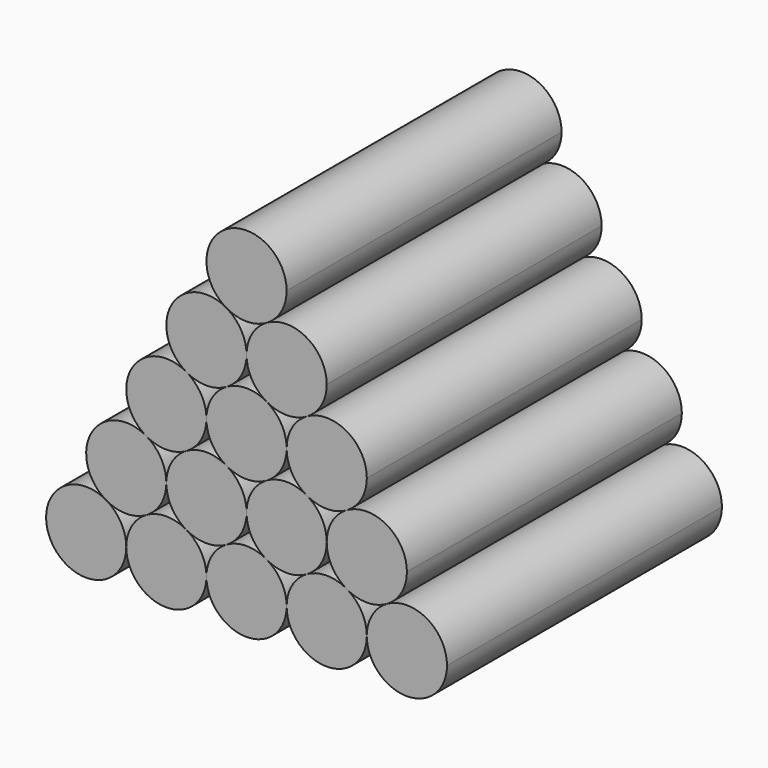
from build123d import *

# Parameters (mm, degrees)
F1_DEPTH = 76.2


# Not quite as in the source:
# - a feature names something its author has since deleted; it is built from what else it names


with BuildPart() as f1:
    # F0 (on Front) → F1 (new body)
    with BuildSketch(Plane.XZ):
        with BuildLine():
            ThreePointArc((-13.3350000199, 23.0968975304), (-25.4789658129, 19.8429317256), (-22.2250001126, 7.6989659046))
            ThreePointArc((-22.2250001126, 7.6989659046), (-17.780000037, 6.5079316793), (-13.3349999515, 7.6989658677))
            ThreePointArc((-13.3349999515, 7.6989658677), (-10.0810341464, 10.9529317035), (-8.89, 15.3979316793))
            ThreePointArc((-8.89, 15.3979316793), (-10.0810341661, 19.8429316893), (-13.3350000199, 23.0968975304))
        make_face()
    extrude(amount=F1_DEPTH)


with BuildPart() as f1b:
    # F0 (on Front) → F1, piece 2 (new body)
    with BuildSketch(Plane.XZ):
        with BuildLine():
            ThreePointArc((-8.89, 15.3979316793), (-7.6989658311, 10.9529316645), (-4.4449999705, 7.6989658226))
            ThreePointArc((-4.4449999705, 7.6989658226), (6.75e-08, 6.5079316793), (4.4450000875, 7.6989658901))
            ThreePointArc((4.4450000875, 7.6989658901), (7.6989658649, 10.952931723), (8.89, 15.3979316793))
            ThreePointArc((8.89, 15.3979316793), (7.6989657927, 19.8429317606), (4.4449998375, 23.0968976128))
            ThreePointArc((4.4449998375, 23.0968976128), (-4.81e-08, 24.2879316793), (-4.4449999207, 23.0968975647))
            ThreePointArc((-4.4449999207, 23.0968975647), (-7.6989658168, 19.8429317189), (-8.89, 15.3979316793))
        make_face()
    extrude(amount=F1_DEPTH)


with BuildPart() as f1c:
    # F0 (on Front) → F1, piece 3 (new body)
    with BuildSketch(Plane.XZ):
        with BuildLine():
            ThreePointArc((8.89, 15.3979316793), (10.0810341244, 10.9529317415), (13.3349998755, 7.6989659115))
            ThreePointArc((13.3349998755, 7.6989659115), (17.7799998064, 6.5079316793), (22.2249997892, 7.6989657179))
            ThreePointArc((22.2249997892, 7.6989657179), (25.4789657788, 10.9529315739), (26.67, 15.3979316793))
            ThreePointArc((26.67, 15.3979316793), (22.2250001076, 23.0968974568), (13.3350002151, 23.0968976431))
            ThreePointArc((13.3350002151, 23.0968976431), (10.0810342225, 19.8429317869), (8.89, 15.3979316793))
        make_face()
    extrude(amount=F1_DEPTH)


with BuildPart() as f1d:
    # F0 (on Front) → F1, piece 4 (new body)
    with BuildSketch(Plane.XZ):
        with BuildLine():
            ThreePointArc((22.2249997892, 7.6989657179), (18.9710340995, 4.4449998946), (17.78, 0))
            ThreePointArc((17.78, 0), (18.9710341607, -4.4450000007), (22.2250000013, -7.6989658404))
            ThreePointArc((22.2250000013, -7.6989658404), (26.6699999179, -8.89), (31.1149998565, -7.6989659225))
            ThreePointArc((31.1149998565, -7.6989659225), (34.3689657982, -4.4450000718), (35.56, 0))
            ThreePointArc((35.56, 0), (31.1149998946, 7.6989659005), (22.2249997892, 7.6989657179))
        make_face()
    extrude(amount=F1_DEPTH)


with BuildPart() as f1e:
    # F0 (on Front) → F1, piece 5 (new body)
    with BuildSketch(Plane.XZ):
        with BuildLine():
            ThreePointArc((4.4450000875, 7.6989658901), (1.1910341856, 4.4450000437), (0, 0))
            ThreePointArc((0, 0), (1.191034094, -4.4449998851), (4.4449997703, -7.698965707))
            ThreePointArc((4.4449997703, -7.698965707), (8.8899998666, -8.89), (13.3349999987, -7.6989658404))
            ThreePointArc((13.3349999987, -7.6989658404), (16.5889658393, -4.4450000007), (17.78, 0))
            ThreePointArc((17.78, 0), (16.5889658037, 4.4450000622), (13.3349998755, 7.6989659115))
            ThreePointArc((13.3349998755, 7.6989659115), (8.8899999786, 8.89), (4.4450000875, 7.6989658901))
        make_face()
    extrude(amount=F1_DEPTH)


with BuildPart() as f1f:
    # F0 (on Front) → F1, piece 6 (new body)
    with BuildSketch(Plane.XZ):
        with BuildLine():
            ThreePointArc((-13.3349999515, 7.6989658677), (-16.5889658256, 4.4450000243), (-17.78, 0))
            ThreePointArc((-17.78, 0), (-16.5889664254, -4.4449989854), (-13.3350020292, -7.6989646681))
            ThreePointArc((-13.3350020292, -7.6989646681), (-8.8900010389, -8.89), (-4.4449997703, -7.698965707))
            ThreePointArc((-4.4449997703, -7.698965707), (-1.191034094, -4.4449998851), (0, 0))
            ThreePointArc((0, 0), (-1.1910341518, 4.4449999853), (-4.4449999705, 7.6989658226))
            ThreePointArc((-4.4449999705, 7.6989658226), (-8.889999955, 8.89), (-13.3349999515, 7.6989658677))
        make_face()
    extrude(amount=F1_DEPTH)


with BuildPart() as f1g:
    # F0 (on Front) → F1, piece 7 (new body)
    with BuildSketch(Plane.XZ):
        with BuildLine():
            ThreePointArc((-22.2249979726, -7.6989646691), (-18.9710335751, -4.4449989863), (-17.78, 0))
            ThreePointArc((-17.78, 0), (-18.9710341928, 4.4450000563), (-22.2250001126, 7.6989659046))
            ThreePointArc((-22.2250001126, 7.6989659046), (-34.3689658547, 4.4449999739), (-31.1150000603, -7.6989658048))
            ThreePointArc((-31.1150000603, -7.6989658048), (-26.6699988643, -8.89), (-22.2249979726, -7.6989646691))
        make_face()
    extrude(amount=F1_DEPTH)


with BuildPart() as f1h:
    # F0 (on Front) → F1, piece 8 (new body)
    with BuildSketch(Plane.XZ):
        with BuildLine():
            ThreePointArc((-26.67, -15.3979316793), (-27.8610341778, -10.9529316492), (-31.1150000603, -7.6989658048))
            ThreePointArc((-31.1150000603, -7.6989658048), (-43.2589658414, -10.9529316824), (-40.0050000541, -23.0968974877))
            ThreePointArc((-40.0050000541, -23.0968974877), (-35.559998118, -24.2879316793), (-31.1149966862, -23.0968956057))
            ThreePointArc((-31.1149966862, -23.0968956057), (-27.8610332037, -19.8429300224), (-26.67, -15.3979316793))
        make_face()
    extrude(amount=F1_DEPTH)


with BuildPart() as f1i:
    # F0 (on Front) → F1, piece 9 (new body)
    with BuildSketch(Plane.XZ):
        with BuildLine():
            ThreePointArc((-13.3350020292, -7.6989646681), (-17.780000001, -6.5079316793), (-22.2249979726, -7.6989646691))
            ThreePointArc((-22.2249979726, -7.6989646691), (-25.4789652544, -10.9529306656), (-26.67, -15.3979316793))
            ThreePointArc((-26.67, -15.3979316793), (-25.4789658625, -19.8429316396), (-22.2250000793, -23.0968974731))
            ThreePointArc((-22.2250000793, -23.0968974731), (-17.7799999131, -24.2879316793), (-13.3349997703, -23.0968973863))
            ThreePointArc((-13.3349997703, -23.0968973863), (-10.081034094, -19.8429315644), (-8.89, -15.3979316793))
            ThreePointArc((-8.89, -15.3979316793), (-10.0810347461, -10.9529306647), (-13.3350020292, -7.6989646681))
        make_face()
    extrude(amount=F1_DEPTH)


with BuildPart() as f1j:
    # F0 (on Front) → F1, piece 10 (new body)
    with BuildSketch(Plane.XZ):
        with BuildLine():
            ThreePointArc((4.4450002297, -7.6989649112), (0, -6.5079306182), (-4.4450002297, -7.6989649112))
            ThreePointArc((-4.4450002297, -7.6989649112), (-7.6989661712, -10.9529311925), (-8.89, -15.3979316793))
            ThreePointArc((-8.89, -15.3979316793), (-7.6989648637, -19.8429323085), (-4.4449975383, -23.0968978791))
            ThreePointArc((-4.4449975383, -23.0968978791), (-6.17e-07, -24.2879306182), (4.4449964696, -23.0968984961))
            ThreePointArc((4.4449964696, -23.0968984961), (7.6989648205, -19.8429323834), (8.89, -15.3979306182))
            ThreePointArc((8.89, -15.3979306182), (7.698965906, -10.9529307331), (4.4450002297, -7.6989649112))
        make_face()
    extrude(amount=F1_DEPTH)


with BuildPart() as f1k:
    # F0 (on Front) → F1, piece 11 (new body)
    with BuildSketch(Plane.XZ):
        with BuildLine():
            ThreePointArc((22.2250000013, -7.6989658404), (17.78, -6.5079316793), (13.3349999987, -7.6989658404))
            ThreePointArc((13.3349999987, -7.6989658404), (10.0810344252, -10.9529312205), (8.89, -15.3979306182))
            ThreePointArc((8.89, -15.3979306182), (10.0810338288, -19.842931105), (13.3349997703, -23.0968973863))
            ThreePointArc((13.3349997703, -23.0968973863), (17.7799999128, -24.2879316793), (22.2250000786, -23.0968974735))
            ThreePointArc((22.2250000786, -23.0968974735), (25.4789658623, -19.84293164), (26.67, -15.3979316793))
            ThreePointArc((26.67, -15.3979316793), (25.47896584, -10.9529316799), (22.2250000013, -7.6989658404))
        make_face()
    extrude(amount=F1_DEPTH)


with BuildPart() as f1l:
    # F0 (on Front) → F1, piece 12 (new body)
    with BuildSketch(Plane.XZ):
        with BuildLine():
            ThreePointArc((44.45, -15.3979316793), (40.0049999282, -7.6989657982), (31.1149998565, -7.6989659225))
            ThreePointArc((31.1149998565, -7.6989659225), (27.8610341189, -10.952931751), (26.67, -15.3979316793))
            ThreePointArc((26.67, -15.3979316793), (27.861034132, -19.8429316301), (31.1149999017, -23.0968974622))
            ThreePointArc((31.1149999017, -23.0968974622), (35.6247538204, -24.2876958462), (40.1166823692, -23.031328419))
            ThreePointArc((40.1166823692, -23.031328419), (43.2911385404, -19.7867352599), (44.45, -15.3979316793))
        make_face()
    extrude(amount=F1_DEPTH)


with BuildPart() as f1m:
    # F0 (on Front) → F1, piece 13 (new body)
    with BuildSketch(Plane.XZ):
        with BuildLine():
            ThreePointArc((-4.4450000175, 38.4948292083), (-16.5889658389, 35.2408633598), (-13.3350000199, 23.0968975304))
            ThreePointArc((-13.3350000199, 23.0968975304), (-8.8899999657, 21.9058633586), (-4.4449999207, 23.0968975647))
            ThreePointArc((-4.4449999207, 23.0968975647), (-1.1910341375, 26.3508633982), (0, 30.7958633586))
            ThreePointArc((0, 30.7958633586), (-1.1910341654, 35.2408633673), (-4.4450000175, 38.4948292083))
        make_face()
    extrude(amount=F1_DEPTH)


with BuildPart() as f1n:
    # F0 (on Front) → F1, piece 14 (new body)
    with BuildSketch(Plane.XZ):
        with BuildLine():
            ThreePointArc((4.4449999987, 38.4948291975), (1.19103416, 35.2408633579), (0, 30.7958633586))
            ThreePointArc((0, 30.7958633586), (1.1910341134, 26.3508634398), (4.4449998375, 23.0968976128))
            ThreePointArc((4.4449998375, 23.0968976128), (8.8900000304, 21.9058633586), (13.3350002151, 23.0968976431))
            ThreePointArc((13.3350002151, 23.0968976431), (16.5889659017, 26.3508634661), (17.78, 30.7958633586))
            ThreePointArc((17.78, 30.7958633586), (13.3349999993, 38.4948291986), (4.4449999987, 38.4948291975))
        make_face()
    extrude(amount=F1_DEPTH)


with BuildPart() as f1o:
    # F0 (on Front) → F1, piece 15 (new body)
    with BuildSketch(Plane.XZ):
        with BuildLine():
            ThreePointArc((8.89, 46.1937950379), (-4.4449999913, 53.8927608825), (-4.4450000175, 38.4948292083))
            ThreePointArc((-4.4450000175, 38.4948292083), (-1.08e-08, 37.3037950379), (4.4449999987, 38.4948291975))
            ThreePointArc((4.4449999987, 38.4948291975), (7.6989658393, 41.7487950372), (8.89, 46.1937950379))
        make_face()
    extrude(amount=F1_DEPTH)


solid = Compound([f1.part, f1b.part, f1c.part, f1d.part, f1e.part, f1f.part, f1g.part, f1h.part, f1i.part, f1j.part, f1k.part, f1l.part, f1m.part, f1n.part, f1o.part])
